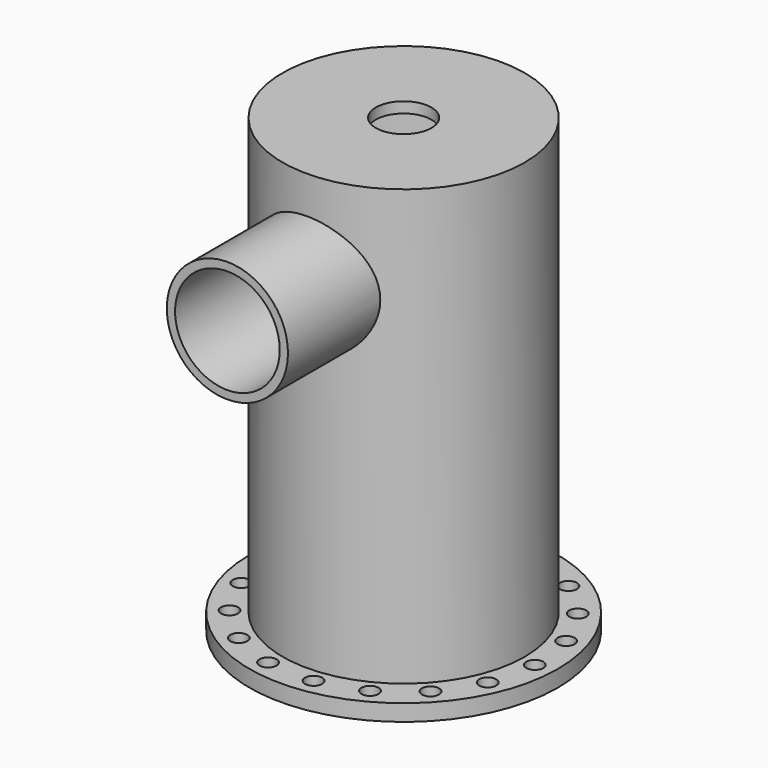
from build123d import *

# Parameters (mm, degrees)
F0_R            = 22
F1_DEPTH        = 82
F2_T            = -1.95
F0_R_2          = 28
F3_DEPTH        = 3
F5_R            = 5.05
F6_DEPTH        = 90
F7_R            = 1.55
F8_DEPTH        = 5
F8_COPIES_COUNT = 18
F10_R           = 11
F12_R           = 9.5
F13_DEPTH       = 30


# Not quite as in the source:
# - a pattern or mirror of a feature is missing from the dataset's text; its kind, count and spacing are read off the source's solid


with BuildPart() as f1:
    # F0 (on Top) → F1 (new body)
    with BuildSketch(Plane.XY):
        Circle(F0_R)
    extrude(amount=F1_DEPTH)

    # F2
    f2_openings = [f1.faces().sort_by_distance(p)[0] for p in [
        (0, 0, 0),
    ]]
    offset(amount=F2_T, openings=f2_openings)

    # F0 (on Top) → F3 (join)
    with BuildSketch(Plane.XY):
        Circle(F0_R_2)
        Circle(F0_R, mode=Mode.SUBTRACT)
    extrude(amount=F3_DEPTH)

    # F5 (on Top) → F6 (cut)
    with BuildSketch(Plane.XY):
        Circle(F5_R)
    extrude(amount=F6_DEPTH, mode=Mode.SUBTRACT)

    # F7 (on face) → F8 (cut)
    with BuildSketch(Plane.XY):
        with Locations((-5.3322692402, -24.1057705134)):
            Circle(F7_R)
    f8 = extrude(amount=F8_DEPTH, mode=Mode.SUBTRACT)

    # F8_copies: F8 ×18 about axis
    f8_copies_axis = Axis((0, 0, 0), (0, 0, 1))
    for i in range(1, F8_COPIES_COUNT):
        add(f8.rotate(f8_copies_axis, i * 360 / F8_COPIES_COUNT), mode=Mode.SUBTRACT)

    # F10 (on offset) → F11 (join, up to the next surface of F1)
    with BuildSketch(Plane.XZ.offset(40)):
        with Locations((0, 64.2171450533)):
            Circle(F10_R)
    extrude(until=Until.NEXT, dir=(0, 1, 0))

    # F12 (on face) → F13 (cut)
    with BuildSketch(Plane.XZ.offset(40)):
        with Locations((0, 64.2171450533)):
            Circle(F12_R)
    extrude(amount=-F13_DEPTH, mode=Mode.SUBTRACT)


solid = f1.part
